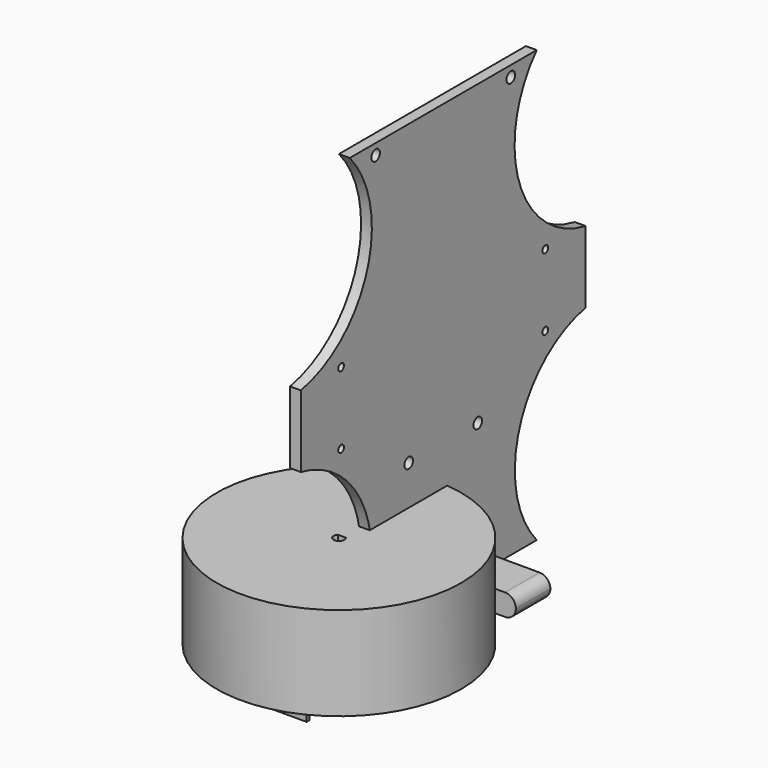
from build123d import *

# Parameters (mm, degrees)
F0_R      = 34
F1_DEPTH  = 26
F3_DEPTH  = 26
F5_DEPTH  = 23
F7_DEPTH  = 10
F9_DEPTH  = 3
F10_W     = 15
F10_H     = 12
F11_DEPTH = 8
F13_DEPTH = 25
F15_DEPTH = 3
F16_W     = 12
F16_H     = 6
F17_DEPTH = 25
F19_R     = 2.99999
F18_R     = 1
F18_R_2   = 1.5
F20_DEPTH = 25


# Not quite as in the source:
# - a fillet or chamfer is up to 0.001 mm smaller than in the source, because OpenCascade refuses the exact size


with BuildPart() as f1:
    # F0 (on Top) → F1 (new body)
    with BuildSketch(Plane.XY):
        Circle(F0_R)
    extrude(amount=F1_DEPTH)

    # F2 (on face) → F3 (cut)
    with BuildSketch(Plane(origin=(0, 0, 0), x_dir=(1, 0, 0), z_dir=(0, 0, -1))):
        with BuildLine():
            Line((-1.1180339887, -1), (1.1180339887, -1))
            ThreePointArc((1.1180339887, -1), (0, 1.5), (-1.1180339887, -1))
        make_face()
    extrude(amount=-F3_DEPTH, mode=Mode.SUBTRACT)


with BuildPart() as f5:
    # F4 (on Top) → F5 (new body)
    with BuildSketch(Plane.XY):
        with BuildLine():
            ThreePointArc((10, 0), (5, 2.75), (0, 0))
            Line((0, 0), (0, -7))
            ThreePointArc((0, -7), (5, -9.75), (10, -7))
            Line((10, -7), (10, 0))
        make_face()
    extrude(amount=F5_DEPTH)

    # F6 (on face) → F7 (join)
    with BuildSketch(Plane(origin=(0, 0, 0), x_dir=(1, 0, 0), z_dir=(0, 0, -1))):
        with BuildLine():
            Line((3.8819660113, 2.5), (6.1180339887, 2.5))
            ThreePointArc((6.1180339887, 2.5), (5, 5), (3.8819660113, 2.5))
        make_face()
    extrude(amount=F7_DEPTH)


with BuildPart() as f9:
    # F8 (on Right) → F9 (new body)
    with BuildSketch(Plane.YZ):
        with BuildLine():
            ThreePointArc((0, -8), (3.5, -4), (0, 0))
            Line((0, 0), (-15, 0))
            ThreePointArc((-15, 0), (-18.5, -4), (-15, -8))
            Line((-15, -8), (-15, -12))
            Line((-15, -12), (0, -12))
            Line((0, -12), (0, -8))
        make_face()
    extrude(amount=F9_DEPTH)

    # F10 (on face) → F11 (join)
    with BuildSketch(Plane(origin=(0, 0, 0), x_dir=(0, -1, 0), z_dir=(-1, 0, 0))):
        with Locations((7.5, -6)):
            Rectangle(F10_W, F10_H)
    extrude(amount=F11_DEPTH)

    # F12 (on face) → F13 (cut)
    with BuildSketch(Plane.XY):
        with BuildLine():
            Line((3, -14), (3, -1))
            Line((3, -1), (-5, -1))
            ThreePointArc((-5, -1), (-6.4142135624, -1.5857864376), (-7, -3))
            Line((-7, -3), (-7, -12))
            ThreePointArc((-7, -12), (-6.4142135624, -13.4142135624), (-5, -14))
            Line((-5, -14), (3, -14))
        make_face()
    extrude(amount=-F13_DEPTH, mode=Mode.SUBTRACT)


with BuildPart() as f15:
    # F14 (on Right) → F15 (new body)
    with BuildSketch(Plane.YZ):
        with BuildLine():
            Line((-17, 70), (-17, 50))
            ThreePointArc((-17, 50), (5.9634758444, 29.9175817871), (0, 0))
            Line((0, 0), (65, 0))
            ThreePointArc((65, 0), (59.0365241556, 29.9175817871), (82, 50))
            Line((82, 50), (82, 70))
            ThreePointArc((82, 70), (58.9246735824, 90.044389018), (65, 120))
            Line((65, 120), (0, 120))
            ThreePointArc((0, 120), (6.0753264176, 90.044389018), (-17, 70))
        make_face()
    extrude(amount=F15_DEPTH)

    # F16 (on face) → F17 (join)
    with BuildSketch(Plane.YZ.offset(3)):
        with Locations((32.5, 7)):
            Rectangle(F16_W, F16_H)
    extrude(amount=F17_DEPTH)

    # F19 (radius 3 in the source; OpenCascade refuses exactly that, so slightly less here)
    f19_edges = [f15.edges().sort_by_distance(p)[0] for p in [
        (28, 32.5, 10),
        (28, 32.5, 4),
    ]]
    fillet(f19_edges, radius=F19_R)

    # F18 (on face) → F20 (cut)
    with BuildSketch(Plane.YZ.offset(3)):
        with Locations((68.0000194097, 50.0062304962)):
            Circle(F18_R)
        with Locations((68.0000194097, 69.9937695038)):
            Circle(F18_R)
        with Locations((-3.0000194097, 50.0062304962)):
            Circle(F18_R)
        with Locations((-3.0000194097, 69.9937695038)):
            Circle(F18_R)
        with Locations((22.5, 7)):
            Circle(F18_R_2)
        with Locations((42.5, 7)):
            Circle(F18_R_2)
        with Locations((9, 117)):
            Circle(F18_R_2)
        with Locations((56, 117)):
            Circle(F18_R_2)
        with Locations((20.4988960177, 37)):
            Circle(F18_R_2)
        with Locations((44.5011039823, 37)):
            Circle(F18_R_2)
    extrude(amount=-F20_DEPTH, mode=Mode.SUBTRACT)


solid = Compound([f1.part, f5.part, f9.part, f15.part])
